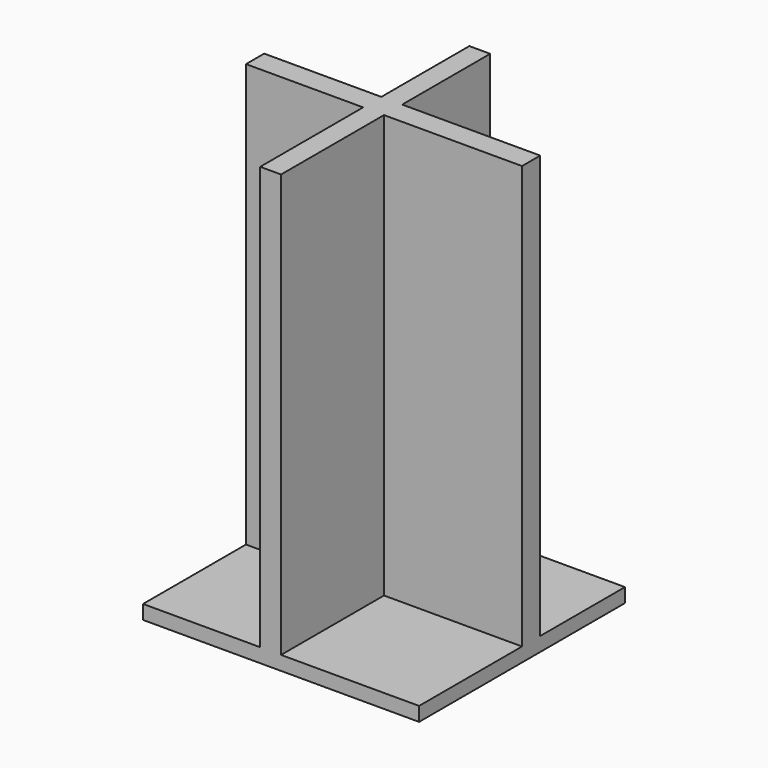
from build123d import *

# Parameters (mm, degrees)
F0_W     = 49.7362613678
F0_H     = 46.3653281331
F1_DEPTH = 2.54
F2_W     = 49.7362613678
F2_H     = 4.098245874
F3_DEPTH = 76.2
F4_W     = 3.7595648319
F4_H     = 23.1826640666
F4_H_2   = 23.9149127156
F5_DEPTH = 76.2


# Not quite as in the source:
# - the program builds the solid bodies; features that only make, move or delete a surface that nothing else refers to are left out


with BuildPart() as f1:
    # F0 (on Top) → F1 (new body)
    with BuildSketch(Plane.XY):
        with Locations((3.7595648319, -4.098245874)):
            Rectangle(F0_W, F0_H)
    extrude(amount=F1_DEPTH)

    # F2 (on face) → F3 (join)
    with BuildSketch(Plane.XY.offset(2.54)):
        with Locations((3.7595648319, -2.049122937)):
            Rectangle(F2_W, F2_H)
    extrude(amount=F3_DEPTH)

    # F4 (on face) → F5 (join)
    with BuildSketch(Plane.XY.offset(2.54)):
        with Locations((1.8797824159, -15.6895779073)):
            Rectangle(F4_W, F4_H)
        with Locations((1.8797824159, 7.8592104837)):
            Rectangle(F4_W, F4_H_2)
    extrude(amount=F5_DEPTH)


solid = f1.part
